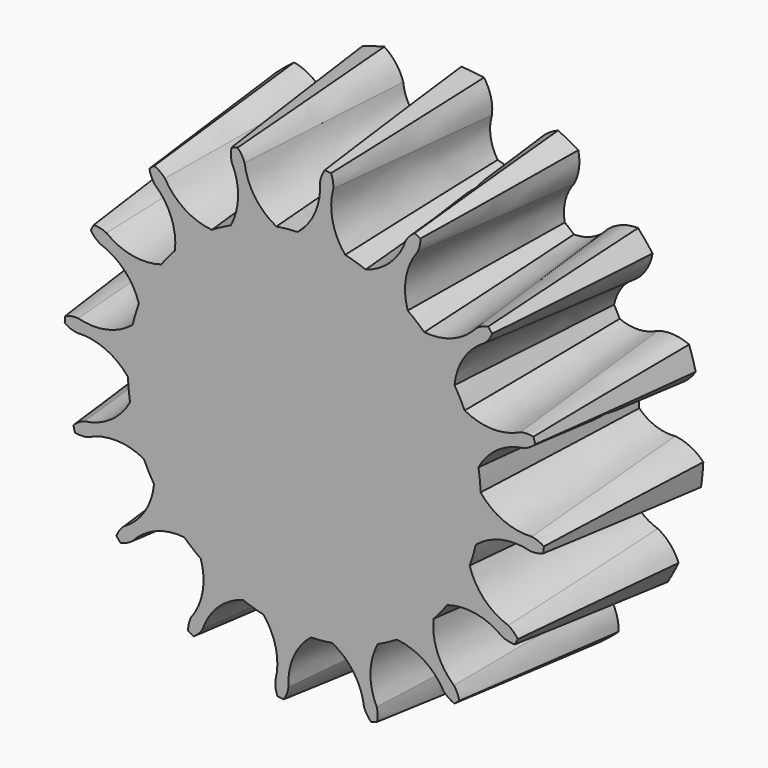
from build123d import *

# Parameters (mm, degrees)
F1_DEPTH               = 254
DRAFT_F1_DRAFTED_ANGLE = 5


# Not quite as in the source:
# - an extrude with a draft is written as a straight extrude whose walls are then drafted


with BuildPart() as f1:
    # F0 (on Front) → F1 (new body)
    with BuildSketch(Plane.XZ):
        with BuildLine():
            ThreePointArc((123.5626635225, 298.306658079), (109.8769987879, 274.1287430978), (87.1719227721, 258.1178557023))
            ThreePointArc((87.1719227721, 258.1178557023), (128.479858706, 240.2429966909), (166.2810782981, 215.8109694899))
            ThreePointArc((166.2810782981, 215.8109694899), (166.9914819537, 243.584415778), (179.5021455508, 268.3907111166))
            ThreePointArc((179.5021455508, 268.3907111166), (186.4313272015, 289.8378529999), (185.424284847, 312.3540542559))
            ThreePointArc((185.424284847, 312.3540542559), (171.302485489, 320.3165295242), (156.8394679821, 327.6409649361))
            ThreePointArc((156.8394679821, 327.6409649361), (137.553364126, 315.9773612323), (123.5626635225, 298.306658079))
        make_face()
        with BuildLine():
            ThreePointArc((298.306658079, 123.5626635225), (271.5330641019, 116.1435222232), (244.1567438337, 120.8770283912))
            ThreePointArc((244.1567438337, 120.8770283912), (260.7264314297, 79.0284727558), (270.1798780284, 35.0229219332))
            ThreePointArc((270.1798780284, 35.0229219332), (290.3210014778, 54.1593828981), (316.7080761946, 62.8537074815))
            ThreePointArc((316.7080761946, 62.8537074815), (336.7731669905, 73.119455611), (351.9824391075, 89.7529006835))
            ThreePointArc((351.9824391075, 89.7529006835), (347.6271392761, 105.3688410293), (342.5793994687, 120.7748967329))
            ThreePointArc((342.5793994687, 120.7748967329), (320.6946513773, 126.1648182802), (298.306658079, 123.5626635225))
        make_face()
        with BuildLine():
            ThreePointArc((228.3140316221, 228.3140316221), (206.4176385925, 211.2138279869), (179.3137822337, 205.1105532468))
            ThreePointArc((179.3137822337, 205.1105532468), (210.6369263738, 172.7884741525), (236.21096743, 135.7503238227))
            ThreePointArc((236.21096743, 135.7503238227), (247.4957325813, 161.1377826862), (268.5470368613, 179.2681875405))
            ThreePointArc((268.5470368613, 179.2681875405), (283.1562318357, 196.4310799397), (290.8424231965, 217.6187158549))
            ThreePointArc((290.8424231965, 217.6187158549), (280.8426891732, 230.3792624329), (270.2835434038, 242.680915579))
            ThreePointArc((270.2835434038, 242.680915579), (248.0020388901, 239.2856232623), (228.3140316221, 228.3140316221))
        make_face()
        with BuildLine():
            ThreePointArc((51.7769800049, 359.5363193931), (35.68303125, 361.4885086721), (19.5180053135, 362.7206474544))
            ThreePointArc((19.5180053135, 362.7206474544), (6.1634365981, 344.5644102965), (0, 322.8848))
            ThreePointArc((0, 322.8848), (-3.3914180447, 295.3100420552), (-18.241071716, 271.8290544714))
            ThreePointArc((-18.241071716, 271.8290544714), (26.7628972231, 271.1227007913), (71.0364023371, 263.0163513836))
            ThreePointArc((71.0364023371, 263.0163513836), (61.0642919802, 288.9475296658), (63.1296797712, 316.6531818931))
            ThreePointArc((63.1296797712, 316.6531818931), (61.3239430051, 339.1194403274), (51.7769800049, 359.5363193931))
        make_face()
        with BuildLine():
            ThreePointArc((-120.8770283912, 244.1567438337), (-79.0284727558, 260.7264314297), (-35.0229219332, 270.1798780284))
            ThreePointArc((-35.0229219332, 270.1798780284), (-54.1593828981, 290.3210014778), (-62.8537074815, 316.7080761946))
            ThreePointArc((-62.8537074815, 316.7080761946), (-73.119455611, 336.7731669905), (-89.7529006835, 351.9824391075))
            ThreePointArc((-89.7529006835, 351.9824391075), (-105.3688410293, 347.6271392761), (-120.7748967329, 342.5793994687))
            ThreePointArc((-120.7748967329, 342.5793994687), (-126.1648182802, 320.6946513773), (-123.5626635225, 298.306658079))
            ThreePointArc((-123.5626635225, 298.306658079), (-116.1435222232, 271.5330641019), (-120.8770283912, 244.1567438337))
        make_face()
        with BuildLine():
            ThreePointArc((-205.1105532468, 179.3137822337), (-172.7884741525, 210.6369263738), (-135.7503238227, 236.21096743))
            ThreePointArc((-135.7503238227, 236.21096743), (-161.1377826862, 247.4957325813), (-179.2681875405, 268.5470368613))
            ThreePointArc((-179.2681875405, 268.5470368613), (-196.4310799397, 283.1562318357), (-217.6187158549, 290.8424231965))
            ThreePointArc((-217.6187158549, 290.8424231965), (-230.3792624329, 280.8426891732), (-242.680915579, 270.2835434038))
            ThreePointArc((-242.680915579, 270.2835434038), (-239.2856232623, 248.0020388901), (-228.3140316221, 228.3140316221))
            ThreePointArc((-228.3140316221, 228.3140316221), (-211.2138279869, 206.4176385925), (-205.1105532468, 179.3137822337))
        make_face()
        with BuildLine():
            ThreePointArc((-258.1178557023, 87.1719227721), (-240.2429966909, 128.479858706), (-215.8109694899, 166.2810782981))
            ThreePointArc((-215.8109694899, 166.2810782981), (-243.584415778, 166.9914819537), (-268.3907111166, 179.5021455508))
            ThreePointArc((-268.3907111166, 179.5021455508), (-289.8378529999, 186.4313272015), (-312.3540542559, 185.424284847))
            ThreePointArc((-312.3540542559, 185.424284847), (-320.3165295242, 171.302485489), (-327.6409649361, 156.8394679821))
            ThreePointArc((-327.6409649361, 156.8394679821), (-315.9773612323, 137.553364126), (-298.306658079, 123.5626635225))
            ThreePointArc((-298.306658079, 123.5626635225), (-274.1287430978, 109.8769987879), (-258.1178557023, 87.1719227721))
        make_face()
        with BuildLine():
            ThreePointArc((-271.8290544714, -18.241071716), (-271.1227007913, 26.7628972231), (-263.0163513836, 71.0364023371))
            ThreePointArc((-263.0163513836, 71.0364023371), (-288.9475296658, 61.0642919802), (-316.6531818931, 63.1296797712))
            ThreePointArc((-316.6531818931, 63.1296797712), (-339.1194403274, 61.3239430051), (-359.5363193931, 51.7769800049))
            ThreePointArc((-359.5363193931, 51.7769800049), (-361.4885086721, 35.68303125), (-362.7206474544, 19.5180053135))
            ThreePointArc((-362.7206474544, 19.5180053135), (-344.5644102965, 6.1634365981), (-322.8848, 0))
            ThreePointArc((-322.8848, 0), (-295.3100420552, -3.3914180447), (-271.8290544714, -18.241071716))
        make_face()
        with BuildLine():
            ThreePointArc((-244.1567438337, -120.8770283912), (-260.7264314297, -79.0284727558), (-270.1798780284, -35.0229219332))
            ThreePointArc((-270.1798780284, -35.0229219332), (-290.3210014778, -54.1593828981), (-316.7080761946, -62.8537074815))
            ThreePointArc((-316.7080761946, -62.8537074815), (-336.7731669905, -73.119455611), (-351.9824391075, -89.7529006835))
            ThreePointArc((-351.9824391075, -89.7529006835), (-347.6271392761, -105.3688410293), (-342.5793994687, -120.7748967329))
            ThreePointArc((-342.5793994687, -120.7748967329), (-320.6946513773, -126.1648182802), (-298.306658079, -123.5626635225))
            ThreePointArc((-298.306658079, -123.5626635225), (-271.5330641019, -116.1435222232), (-244.1567438337, -120.8770283912))
        make_face()
        with BuildLine():
            ThreePointArc((-179.3137822337, -205.1105532468), (-210.6369263738, -172.7884741525), (-236.21096743, -135.7503238227))
            ThreePointArc((-236.21096743, -135.7503238227), (-247.4957325813, -161.1377826862), (-268.5470368613, -179.2681875405))
            ThreePointArc((-268.5470368613, -179.2681875405), (-283.1562318357, -196.4310799397), (-290.8424231965, -217.6187158549))
            ThreePointArc((-290.8424231965, -217.6187158549), (-280.8426891732, -230.3792624329), (-270.2835434038, -242.680915579))
            ThreePointArc((-270.2835434038, -242.680915579), (-248.0020388901, -239.2856232623), (-228.3140316221, -228.3140316221))
            ThreePointArc((-228.3140316221, -228.3140316221), (-206.4176385925, -211.2138279869), (-179.3137822337, -205.1105532468))
        make_face()
        with BuildLine():
            ThreePointArc((-87.1719227721, -258.1178557023), (-128.479858706, -240.2429966909), (-166.2810782981, -215.8109694899))
            ThreePointArc((-166.2810782981, -215.8109694899), (-166.9914819537, -243.584415778), (-179.5021455508, -268.3907111166))
            ThreePointArc((-179.5021455508, -268.3907111166), (-186.4313272015, -289.8378529999), (-185.424284847, -312.3540542559))
            ThreePointArc((-185.424284847, -312.3540542559), (-171.302485489, -320.3165295242), (-156.8394679821, -327.6409649361))
            ThreePointArc((-156.8394679821, -327.6409649361), (-137.553364126, -315.9773612323), (-123.5626635225, -298.306658079))
            ThreePointArc((-123.5626635225, -298.306658079), (-109.8769987879, -274.1287430978), (-87.1719227721, -258.1178557023))
        make_face()
        with BuildLine():
            ThreePointArc((18.241071716, -271.8290544714), (-26.7628972231, -271.1227007913), (-71.0364023371, -263.0163513836))
            ThreePointArc((-71.0364023371, -263.0163513836), (-61.0642919802, -288.9475296658), (-63.1296797712, -316.6531818931))
            ThreePointArc((-63.1296797712, -316.6531818931), (-61.3239430051, -339.1194403274), (-51.7769800049, -359.5363193931))
            ThreePointArc((-51.7769800049, -359.5363193931), (-35.68303125, -361.4885086721), (-19.5180053135, -362.7206474544))
            ThreePointArc((-19.5180053135, -362.7206474544), (-6.1634365981, -344.5644102965), (0, -322.8848))
            ThreePointArc((0, -322.8848), (3.3914180447, -295.3100420552), (18.241071716, -271.8290544714))
        make_face()
        with BuildLine():
            ThreePointArc((123.5626635225, -298.306658079), (116.1435222232, -271.5330641019), (120.8770283912, -244.1567438337))
            ThreePointArc((120.8770283912, -244.1567438337), (79.0284727558, -260.7264314297), (35.0229219332, -270.1798780284))
            ThreePointArc((35.0229219332, -270.1798780284), (54.1593828981, -290.3210014778), (62.8537074815, -316.7080761946))
            ThreePointArc((62.8537074815, -316.7080761946), (73.119455611, -336.7731669905), (89.7529006835, -351.9824391075))
            ThreePointArc((89.7529006835, -351.9824391075), (105.3688410293, -347.6271392761), (120.7748967329, -342.5793994687))
            ThreePointArc((120.7748967329, -342.5793994687), (126.1648182802, -320.6946513773), (123.5626635225, -298.306658079))
        make_face()
        with BuildLine():
            ThreePointArc((228.3140316221, -228.3140316221), (211.2138279869, -206.4176385925), (205.1105532468, -179.3137822337))
            ThreePointArc((205.1105532468, -179.3137822337), (172.7884741525, -210.6369263738), (135.7503238227, -236.21096743))
            ThreePointArc((135.7503238227, -236.21096743), (161.1377826862, -247.4957325813), (179.2681875405, -268.5470368613))
            ThreePointArc((179.2681875405, -268.5470368613), (196.4310799397, -283.1562318357), (217.6187158549, -290.8424231965))
            ThreePointArc((217.6187158549, -290.8424231965), (230.3792624329, -280.8426891732), (242.680915579, -270.2835434038))
            ThreePointArc((242.680915579, -270.2835434038), (239.2856232623, -248.0020388901), (228.3140316221, -228.3140316221))
        make_face()
        with BuildLine():
            ThreePointArc((298.306658079, -123.5626635225), (274.1287430978, -109.8769987879), (258.1178557023, -87.1719227721))
            ThreePointArc((258.1178557023, -87.1719227721), (240.2429966909, -128.479858706), (215.8109694899, -166.2810782981))
            ThreePointArc((215.8109694899, -166.2810782981), (243.584415778, -166.9914819537), (268.3907111166, -179.5021455508))
            ThreePointArc((268.3907111166, -179.5021455508), (289.8378529999, -186.4313272015), (312.3540542559, -185.424284847))
            ThreePointArc((312.3540542559, -185.424284847), (320.3165295242, -171.302485489), (327.6409649361, -156.8394679821))
            ThreePointArc((327.6409649361, -156.8394679821), (315.9773612323, -137.553364126), (298.306658079, -123.5626635225))
        make_face()
        with BuildLine():
            ThreePointArc((322.8848, 0), (295.3100420552, 3.3914180447), (271.8290544714, 18.241071716))
            ThreePointArc((271.8290544714, 18.241071716), (272.2875207239, 9.1256566984), (272.4404, 0))
            ThreePointArc((272.4404, 0), (270.0741116154, -35.8293983668), (263.0163513836, -71.0364023371))
            ThreePointArc((263.0163513836, -71.0364023371), (288.9475296658, -61.0642919802), (316.6531818931, -63.1296797712))
            ThreePointArc((316.6531818931, -63.1296797712), (339.1194403274, -61.3239430051), (359.5363193931, -51.7769800049))
            ThreePointArc((359.5363193931, -51.7769800049), (361.4885086721, -35.68303125), (362.7206474544, -19.5180053135))
            ThreePointArc((362.7206474544, -19.5180053135), (344.5644102965, -6.1634365981), (322.8848, 0))
        make_face()
        with BuildLine():
            ThreePointArc((71.0364023371, 263.0163513836), (26.7628972231, 271.1227007913), (-18.241071716, 271.8290544714))
            ThreePointArc((-18.241071716, 271.8290544714), (-26.6447593459, 271.1343363566), (-35.0229219332, 270.1798780284))
            ThreePointArc((-35.0229219332, 270.1798780284), (-79.0284727558, 260.7264314297), (-120.8770283912, 244.1567438337))
            ThreePointArc((-120.8770283912, 244.1567438337), (-128.3751662774, 240.2989559599), (-135.7503238227, 236.21096743))
            ThreePointArc((-135.7503238227, 236.21096743), (-172.7884741525, 210.6369263738), (-205.1105532468, 179.3137822337))
            ThreePointArc((-205.1105532468, 179.3137822337), (-210.5616178669, 172.8802378337), (-215.8109694899, 166.2810782981))
            ThreePointArc((-215.8109694899, 166.2810782981), (-240.2429966909, 128.479858706), (-258.1178557023, 87.1719227721))
            ThreePointArc((-258.1178557023, 87.1719227721), (-260.691971882, 79.1420706606), (-263.0163513836, 71.0364023371))
            ThreePointArc((-263.0163513836, 71.0364023371), (-271.1227007913, 26.7628972231), (-271.8290544714, -18.241071716))
            ThreePointArc((-271.8290544714, -18.241071716), (-271.1343363566, -26.6447593459), (-270.1798780284, -35.0229219332))
            ThreePointArc((-270.1798780284, -35.0229219332), (-260.7264314297, -79.0284727558), (-244.1567438337, -120.8770283912))
            ThreePointArc((-244.1567438337, -120.8770283912), (-240.2989559599, -128.3751662774), (-236.21096743, -135.7503238227))
            ThreePointArc((-236.21096743, -135.7503238227), (-210.6369263738, -172.7884741525), (-179.3137822337, -205.1105532468))
            ThreePointArc((-179.3137822337, -205.1105532468), (-172.8802378337, -210.5616178669), (-166.2810782981, -215.8109694899))
            ThreePointArc((-166.2810782981, -215.8109694899), (-128.479858706, -240.2429966909), (-87.1719227721, -258.1178557023))
            ThreePointArc((-87.1719227721, -258.1178557023), (-79.1420706606, -260.691971882), (-71.0364023371, -263.0163513836))
            ThreePointArc((-71.0364023371, -263.0163513836), (-26.7628972231, -271.1227007913), (18.241071716, -271.8290544714))
            ThreePointArc((18.241071716, -271.8290544714), (26.6447593459, -271.1343363566), (35.0229219332, -270.1798780284))
            ThreePointArc((35.0229219332, -270.1798780284), (79.0284727558, -260.7264314297), (120.8770283912, -244.1567438337))
            ThreePointArc((120.8770283912, -244.1567438337), (128.3751662774, -240.2989559599), (135.7503238227, -236.21096743))
            ThreePointArc((135.7503238227, -236.21096743), (172.7884741525, -210.6369263738), (205.1105532468, -179.3137822337))
            ThreePointArc((205.1105532468, -179.3137822337), (210.5616178669, -172.8802378337), (215.8109694899, -166.2810782981))
            ThreePointArc((215.8109694899, -166.2810782981), (240.2429966909, -128.479858706), (258.1178557023, -87.1719227721))
            ThreePointArc((258.1178557023, -87.1719227721), (260.691971882, -79.1420706606), (263.0163513836, -71.0364023371))
            ThreePointArc((263.0163513836, -71.0364023371), (270.0741116154, -35.8293983668), (272.4404, 0))
            ThreePointArc((272.4404, 0), (272.2875207239, 9.1256566984), (271.8290544714, 18.241071716))
            ThreePointArc((271.8290544714, 18.241071716), (271.1343363566, 26.6447593459), (270.1798780284, 35.0229219332))
            ThreePointArc((270.1798780284, 35.0229219332), (260.7264314297, 79.0284727558), (244.1567438337, 120.8770283912))
            ThreePointArc((244.1567438337, 120.8770283912), (240.2989559599, 128.3751662774), (236.21096743, 135.7503238227))
            ThreePointArc((236.21096743, 135.7503238227), (210.6369263738, 172.7884741525), (179.3137822337, 205.1105532468))
            ThreePointArc((179.3137822337, 205.1105532468), (172.8802378337, 210.5616178669), (166.2810782981, 215.8109694899))
            ThreePointArc((166.2810782981, 215.8109694899), (128.479858706, 240.2429966909), (87.1719227721, 258.1178557023))
            ThreePointArc((87.1719227721, 258.1178557023), (79.1420706606, 260.691971882), (71.0364023371, 263.0163513836))
        make_face()
    extrude(amount=F1_DEPTH)

    # draft_F1_drafted
    draft_f1_drafted_walls = [f1.faces().sort_by_distance(p)[0] for p in [
        (137.553364126, -169.3333333333, 315.9773612323),
        (109.8769987879, -169.3333333333, 274.1287430978),
        (79.1420706606, -169.3333333333, 260.691971882),
        (61.0642919802, -169.3333333333, 288.9475296658),
        (61.3239430051, -169.3333333333, 339.1194403274),
        (35.68303125, -169.3333333333, 361.4885086721),
        (6.1634365981, -169.3333333333, 344.5644102965),
        (-3.3914180447, -169.3333333333, 295.3100420552),
        (-26.6447593459, -169.3333333333, 271.1343363566),
        (-54.1593828981, -169.3333333333, 290.3210014778),
        (-73.119455611, -169.3333333333, 336.7731669905),
        (-105.3688410293, -169.3333333333, 347.6271392761),
        (-126.1648182802, -169.3333333333, 320.6946513773),
        (-116.1435222232, -169.3333333333, 271.5330641019),
        (-128.3751662774, -169.3333333333, 240.2989559599),
        (-161.1377826862, -169.3333333333, 247.4957325813),
        (-196.4310799397, -169.3333333333, 283.1562318357),
        (-230.3792624329, -169.3333333333, 280.8426891732),
        (-239.2856232623, -169.3333333333, 248.0020388901),
        (-211.2138279869, -169.3333333333, 206.4176385925),
        (-210.5616178669, -169.3333333333, 172.8802378337),
        (-243.584415778, -169.3333333333, 166.9914819537),
        (-289.8378529999, -169.3333333333, 186.4313272015),
        (-320.3165295242, -169.3333333333, 171.302485489),
        (-315.9773612323, -169.3333333333, 137.553364126),
        (-274.1287430978, -169.3333333333, 109.8769987879),
        (-260.691971882, -169.3333333333, 79.1420706606),
        (-288.9475296658, -169.3333333333, 61.0642919802),
        (-339.1194403274, -169.3333333333, 61.3239430051),
        (-361.4885086721, -169.3333333333, 35.68303125),
        (-344.5644102965, -169.3333333333, 6.1634365981),
        (-295.3100420552, -169.3333333333, -3.3914180447),
        (-271.1343363566, -169.3333333333, -26.6447593459),
        (-290.3210014778, -169.3333333333, -54.1593828981),
        (-336.7731669905, -169.3333333333, -73.119455611),
        (-347.6271392761, -169.3333333333, -105.3688410293),
        (-320.6946513773, -169.3333333333, -126.1648182802),
        (-271.5330641019, -169.3333333333, -116.1435222232),
        (-240.2989559599, -169.3333333333, -128.3751662774),
        (-247.4957325813, -169.3333333333, -161.1377826862),
        (-283.1562318357, -169.3333333333, -196.4310799397),
        (-280.8426891732, -169.3333333333, -230.3792624329),
        (-248.0020388901, -169.3333333333, -239.2856232623),
        (-206.4176385925, -169.3333333333, -211.2138279869),
        (-172.8802378337, -169.3333333333, -210.5616178669),
        (-166.9914819537, -169.3333333333, -243.584415778),
        (-186.4313272015, -169.3333333333, -289.8378529999),
        (-171.302485489, -169.3333333333, -320.3165295242),
        (-137.553364126, -169.3333333333, -315.9773612323),
        (-109.8769987879, -169.3333333333, -274.1287430978),
        (-79.1420706606, -169.3333333333, -260.691971882),
        (-61.0642919802, -169.3333333333, -288.9475296658),
        (-61.3239430051, -169.3333333333, -339.1194403274),
        (-35.68303125, -169.3333333333, -361.4885086721),
        (-6.1634365981, -169.3333333333, -344.5644102965),
        (3.3914180447, -169.3333333333, -295.3100420552),
        (26.6447593459, -169.3333333333, -271.1343363566),
        (54.1593828981, -169.3333333333, -290.3210014778),
        (73.119455611, -169.3333333333, -336.7731669905),
        (105.3688410293, -169.3333333333, -347.6271392761),
        (126.1648182802, -169.3333333333, -320.6946513773),
        (116.1435222232, -169.3333333333, -271.5330641019),
        (128.3751662774, -169.3333333333, -240.2989559599),
        (161.1377826862, -169.3333333333, -247.4957325813),
        (196.4310799397, -169.3333333333, -283.1562318357),
        (230.3792624329, -169.3333333333, -280.8426891732),
        (239.2856232623, -169.3333333333, -248.0020388901),
        (211.2138279869, -169.3333333333, -206.4176385925),
        (210.5616178669, -169.3333333333, -172.8802378337),
        (243.584415778, -169.3333333333, -166.9914819537),
        (289.8378529999, -169.3333333333, -186.4313272015),
        (320.3165295242, -169.3333333333, -171.302485489),
        (315.9773612323, -169.3333333333, -137.553364126),
        (274.1287430978, -169.3333333333, -109.8769987879),
        (260.691971882, -169.3333333333, -79.1420706606),
        (288.9475296658, -169.3333333333, -61.0642919802),
        (339.1194403274, -169.3333333333, -61.3239430051),
        (361.4885086721, -169.3333333333, -35.68303125),
        (344.5644102965, -169.3333333333, -6.1634365981),
        (295.3100420552, -169.3333333333, 3.3914180447),
        (271.1343363566, -169.3333333333, 26.6447593459),
        (290.3210014778, -169.3333333333, 54.1593828981),
        (336.7731669905, -169.3333333333, 73.119455611),
        (347.6271392761, -169.3333333333, 105.3688410293),
        (320.6946513773, -169.3333333333, 126.1648182802),
        (271.5330641019, -169.3333333333, 116.1435222232),
        (240.2989559599, -169.3333333333, 128.3751662774),
        (247.4957325813, -169.3333333333, 161.1377826862),
        (283.1562318357, -169.3333333333, 196.4310799397),
        (280.8426891732, -169.3333333333, 230.3792624329),
        (248.0020388901, -169.3333333333, 239.2856232623),
        (206.4176385925, -169.3333333333, 211.2138279869),
        (172.8802378337, -169.3333333333, 210.5616178669),
        (166.9914819537, -169.3333333333, 243.584415778),
        (186.4313272015, -169.3333333333, 289.8378529999),
        (171.302485489, -169.3333333333, 320.3165295242),
    ]]
    draft(draft_f1_drafted_walls, neutral_plane=Plane.XZ, angle=DRAFT_F1_DRAFTED_ANGLE)


solid = f1.part
